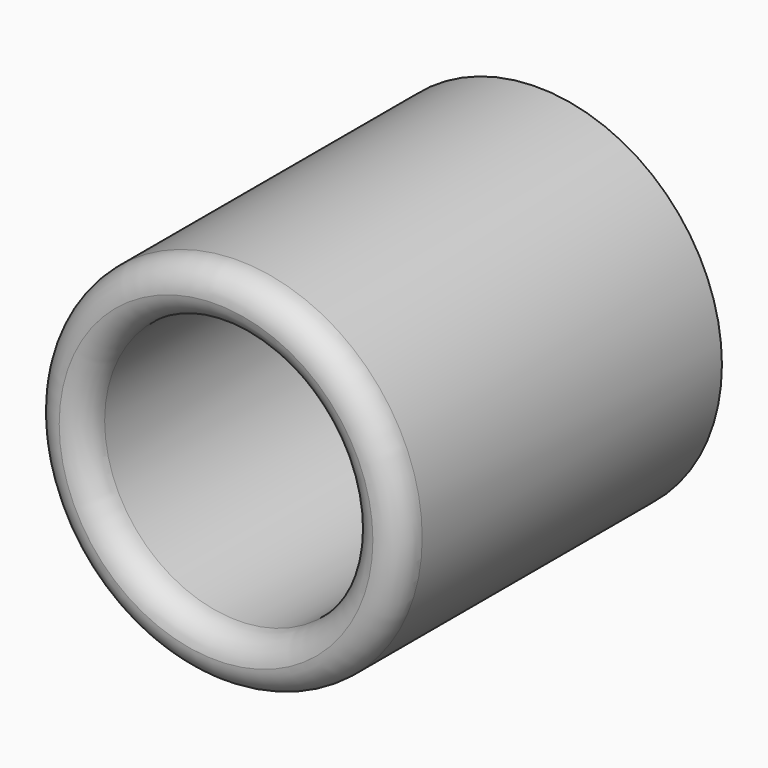
from build123d import *

# Parameters (mm, degrees)
F0_R     = 33.6400886769
F0_R_2   = 24.263041798
F1_DEPTH = 73.4
F2_R     = 5


# Not quite as in the source:
# - a fillet or chamfer that OpenCascade refuses, or shapes differently, is made with other operations: its cross-section is extruded or revolved along the edge and cut away or added


with BuildPart() as f1:
    # F0 (on Front) → F1 (new body)
    with BuildSketch(Plane.XZ):
        with Locations((-20.8813920617, 29.2152203619)):
            Circle(F0_R)
        with Locations((-20.8813920617, 29.2152203619)):
            Circle(F0_R_2, mode=Mode.SUBTRACT)
    extrude(amount=F1_DEPTH)

    # F2
    f2_edges = [f1.edges().sort_by_distance(p)[0] for p in [
        (-54.521481, -73.4, 29.21522),
    ]]
    fillet(f2_edges, radius=F2_R)

    # F3: fillet of radius 5 on 1 edges, made by hand

    # F3_s1 → F3_t2 (revolve, cut)
    with BuildSketch(Plane.XY.offset(29.2152203619)):
        with BuildLine():
            ThreePointArc((7.7586467113, -73.4003968748), (4.6319918458, -71.7466536397), (3.3812497363, -68.4381069026))
            Line((3.3812497363, -68.4381069026), (2.8811131677, -68.4381069026))
            ThreePointArc((2.8811131677, -68.4381069026), (2.8815131677, -70.9190534513), (2.8815131677, -73.4))
            Line((2.8815131677, -73.4), (3.3816497363, -73.9001365685))
            ThreePointArc((3.3816497363, -73.9001365685), (5.5701482238, -73.9001365685), (7.6962498403, -73.896625872))
            Line((7.6962498403, -73.896625872), (7.7586467113, -73.4003968748))
        make_face()
    revolve(axis=Axis((-20.8813920617, -73.4, 29.2152203619), (0, -1, 0)), mode=Mode.SUBTRACT)


solid = f1.part
